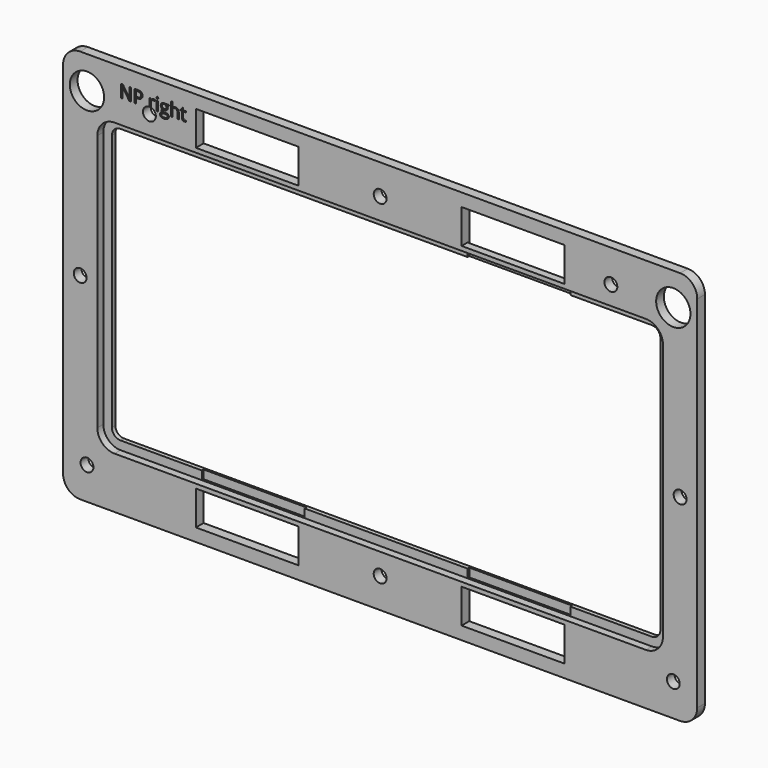
from build123d import *

# Parameters (mm, degrees)
F0_R         = 2.38125
F0_W         = 38.1
F0_H         = 12.7
F0_R_2       = 6.35
F0_R_3       = 2.3876
F1_DEPTH     = 0.79375
F3_DEPTH     = 3.571875
F4_W         = 38.1
F4_H         = 6.4444152495
F4_H_2       = 7.2760339895
F5_DEPTH     = 0.79375
F6_DEPTH     = 0.79375
F7_TEXT_SIZE = 6.5434620612
F8_DEPTH     = 0.396875


# Not quite as in the source:
# - Text() gives the source's letters only with a copy of the font that has no kerning and outlines rounded to 1/6400 em; it was checked with that copy


with BuildPart() as f1:
    # F0 (on Front) → F1 (new body)
    with BuildSketch(Plane.XZ):
        with BuildLine():
            Line((58.8975986641, 62.01647109), (-163.3524013359, 62.01647109))
            ThreePointArc((-163.3524013359, 62.01647109), (-167.8425293965, 60.1565991505), (-169.7024013359, 55.66647109))
            Line((-169.7024013359, 55.66647109), (-169.7024013359, -77.68352891))
            ThreePointArc((-169.7024013359, -77.68352891), (-167.8425293965, -82.1736569705), (-163.3524013359, -84.03352891))
            Line((-163.3524013359, -84.03352891), (58.8975986641, -84.03352891))
            ThreePointArc((58.8975986641, -84.03352891), (63.3877267246, -82.1736569705), (65.2475986641, -77.68352891))
            Line((65.2475986641, -77.68352891), (65.2475986641, 55.66647109))
            ThreePointArc((65.2475986641, 55.66647109), (63.3877267246, 60.1565991505), (58.8975986641, 62.01647109))
        make_face()
        with Locations((-160.8349653662, -71.9910929403)):
            Circle(F0_R, mode=Mode.SUBTRACT)
        with Locations((-101.4399013359, -72.92102891)):
            Rectangle(F0_W, F0_H, mode=Mode.SUBTRACT)
        with Locations((-52.2274013359, -72.92102891)):
            Circle(F0_R, mode=Mode.SUBTRACT)
        with Locations((-3.0149013359, -72.92102891)):
            Rectangle(F0_W, F0_H, mode=Mode.SUBTRACT)
        with Locations((56.3801626943, -71.9910929403)):
            Circle(F0_R, mode=Mode.SUBTRACT)
        with Locations((-163.3524013359, -11.00852891)):
            Circle(F0_R, mode=Mode.SUBTRACT)
        with BuildLine():
            ThreePointArc((-157.0024013359, 36.61647109), (-155.1425293965, 41.1065991505), (-150.6524013359, 42.96647109))
            Line((-150.6524013359, 42.96647109), (46.1975986641, 42.96647109))
            ThreePointArc((46.1975986641, 42.96647109), (50.6877267246, 41.1065991505), (52.5475986641, 36.61647109))
            Line((52.5475986641, 36.61647109), (52.5475986641, -58.63352891))
            ThreePointArc((52.5475986641, -58.63352891), (50.6877267246, -63.1236569705), (46.1975986641, -64.98352891))
            Line((46.1975986641, -64.98352891), (-150.6524013359, -64.98352891))
            ThreePointArc((-150.6524013359, -64.98352891), (-155.1425293965, -63.1236569705), (-157.0024013359, -58.63352891))
            Line((-157.0024013359, -58.63352891), (-157.0024013359, 36.61647109))
        make_face(mode=Mode.SUBTRACT)
        with Locations((-160.8349653662, 49.9740351203)):
            Circle(F0_R_2, mode=Mode.SUBTRACT)
        with Locations((-137.7049037359, 49.9740351203)):
            Circle(F0_R_3, mode=Mode.SUBTRACT)
        with Locations((-101.4399013359, 50.90397109)):
            Rectangle(F0_W, F0_H, mode=Mode.SUBTRACT)
        with Locations((-52.2274013359, 50.90397109)):
            Circle(F0_R, mode=Mode.SUBTRACT)
        with Locations((58.8975986641, -11.00852891)):
            Circle(F0_R, mode=Mode.SUBTRACT)
        with Locations((-3.0149013359, 50.90397109)):
            Rectangle(F0_W, F0_H, mode=Mode.SUBTRACT)
        with Locations((33.2501010641, 49.9740351203)):
            Circle(F0_R_3, mode=Mode.SUBTRACT)
        with Locations((56.3801626943, 49.9740351203)):
            Circle(F0_R_2, mode=Mode.SUBTRACT)
        with BuildLine():
            Line((46.1975986641, 42.96647109), (-150.6524013359, 42.96647109))
            ThreePointArc((-150.6524013359, 42.96647109), (-155.1425293965, 41.1065991505), (-157.0024013359, 36.61647109))
            Line((-157.0024013359, 36.61647109), (-157.0024013359, -58.63352891))
            ThreePointArc((-157.0024013359, -58.63352891), (-155.1425293965, -63.1236569705), (-150.6524013359, -64.98352891))
            Line((-150.6524013359, -64.98352891), (46.1975986641, -64.98352891))
            ThreePointArc((46.1975986641, -64.98352891), (50.6877267246, -63.1236569705), (52.5475986641, -58.63352891))
            Line((52.5475986641, -58.63352891), (52.5475986641, 36.61647109))
            ThreePointArc((52.5475986641, 36.61647109), (50.6877267246, 41.1065991505), (46.1975986641, 42.96647109))
        make_face()
        with BuildLine():
            ThreePointArc((-153.8274013359, 36.61647109), (-152.8974653662, 38.8615351203), (-150.6524013359, 39.79147109))
            Line((-150.6524013359, 39.79147109), (46.1975986641, 39.79147109))
            ThreePointArc((46.1975986641, 39.79147109), (48.4426626943, 38.8615351203), (49.3725986641, 36.61647109))
            Line((49.3725986641, 36.61647109), (49.3725986641, -58.63352891))
            ThreePointArc((49.3725986641, -58.63352891), (48.4426626943, -60.8785929403), (46.1975986641, -61.80852891))
            Line((46.1975986641, -61.80852891), (-150.6524013359, -61.80852891))
            ThreePointArc((-150.6524013359, -61.80852891), (-152.8974653662, -60.8785929403), (-153.8274013359, -58.63352891))
            Line((-153.8274013359, -58.63352891), (-153.8274013359, 36.61647109))
        make_face(mode=Mode.SUBTRACT)
    extrude(amount=F1_DEPTH)

    # F0 (on Front) → F3 (join)
    with BuildSketch(Plane.XZ):
        with BuildLine():
            Line((58.8975986641, 62.01647109), (-163.3524013359, 62.01647109))
            ThreePointArc((-163.3524013359, 62.01647109), (-167.8425293965, 60.1565991505), (-169.7024013359, 55.66647109))
            Line((-169.7024013359, 55.66647109), (-169.7024013359, -77.68352891))
            ThreePointArc((-169.7024013359, -77.68352891), (-167.8425293965, -82.1736569705), (-163.3524013359, -84.03352891))
            Line((-163.3524013359, -84.03352891), (58.8975986641, -84.03352891))
            ThreePointArc((58.8975986641, -84.03352891), (63.3877267246, -82.1736569705), (65.2475986641, -77.68352891))
            Line((65.2475986641, -77.68352891), (65.2475986641, 55.66647109))
            ThreePointArc((65.2475986641, 55.66647109), (63.3877267246, 60.1565991505), (58.8975986641, 62.01647109))
        make_face()
        with Locations((-160.8349653662, -71.9910929403)):
            Circle(F0_R, mode=Mode.SUBTRACT)
        with Locations((-101.4399013359, -72.92102891)):
            Rectangle(F0_W, F0_H, mode=Mode.SUBTRACT)
        with Locations((-52.2274013359, -72.92102891)):
            Circle(F0_R, mode=Mode.SUBTRACT)
        with Locations((-3.0149013359, -72.92102891)):
            Rectangle(F0_W, F0_H, mode=Mode.SUBTRACT)
        with Locations((56.3801626943, -71.9910929403)):
            Circle(F0_R, mode=Mode.SUBTRACT)
        with Locations((-163.3524013359, -11.00852891)):
            Circle(F0_R, mode=Mode.SUBTRACT)
        with BuildLine():
            ThreePointArc((-157.0024013359, 36.61647109), (-155.1425293965, 41.1065991505), (-150.6524013359, 42.96647109))
            Line((-150.6524013359, 42.96647109), (46.1975986641, 42.96647109))
            ThreePointArc((46.1975986641, 42.96647109), (50.6877267246, 41.1065991505), (52.5475986641, 36.61647109))
            Line((52.5475986641, 36.61647109), (52.5475986641, -58.63352891))
            ThreePointArc((52.5475986641, -58.63352891), (50.6877267246, -63.1236569705), (46.1975986641, -64.98352891))
            Line((46.1975986641, -64.98352891), (-150.6524013359, -64.98352891))
            ThreePointArc((-150.6524013359, -64.98352891), (-155.1425293965, -63.1236569705), (-157.0024013359, -58.63352891))
            Line((-157.0024013359, -58.63352891), (-157.0024013359, 36.61647109))
        make_face(mode=Mode.SUBTRACT)
        with Locations((-160.8349653662, 49.9740351203)):
            Circle(F0_R_2, mode=Mode.SUBTRACT)
        with Locations((-137.7049037359, 49.9740351203)):
            Circle(F0_R_3, mode=Mode.SUBTRACT)
        with Locations((-101.4399013359, 50.90397109)):
            Rectangle(F0_W, F0_H, mode=Mode.SUBTRACT)
        with Locations((-52.2274013359, 50.90397109)):
            Circle(F0_R, mode=Mode.SUBTRACT)
        with Locations((58.8975986641, -11.00852891)):
            Circle(F0_R, mode=Mode.SUBTRACT)
        with Locations((-3.0149013359, 50.90397109)):
            Rectangle(F0_W, F0_H, mode=Mode.SUBTRACT)
        with Locations((33.2501010641, 49.9740351203)):
            Circle(F0_R_3, mode=Mode.SUBTRACT)
        with Locations((56.3801626943, 49.9740351203)):
            Circle(F0_R_2, mode=Mode.SUBTRACT)
    extrude(amount=F3_DEPTH)

    # F4 (on face) → F5 (cut)
    with BuildSketch(Plane(origin=(0, 0, 0), x_dir=(-1, 0, 0), z_dir=(0, 1, 0))):
        with Locations((3.0149013359, 41.3317634652)):
            Rectangle(F4_W, F4_H)
        with Locations((3.0149013359, -62.9330119152)):
            Rectangle(F4_W, F4_H_2)
        with Locations((101.4399013359, -62.9330119152)):
            Rectangle(F4_W, F4_H_2)
    extrude(amount=-F5_DEPTH, mode=Mode.SUBTRACT)

    # F2 (on face) → F6 (join)
    with BuildSketch(Plane.XZ):
        with BuildLine():
            Line((46.1975986641, 42.96647109), (-150.6524013359, 42.96647109))
            ThreePointArc((-150.6524013359, 42.96647109), (-155.1425293965, 41.1065991505), (-157.0024013359, 36.61647109))
            Line((-157.0024013359, 36.61647109), (-157.0024013359, -58.63352891))
            ThreePointArc((-157.0024013359, -58.63352891), (-155.1425293965, -63.1236569705), (-150.6524013359, -64.98352891))
            Line((-150.6524013359, -64.98352891), (46.1975986641, -64.98352891))
            ThreePointArc((46.1975986641, -64.98352891), (50.6877267246, -63.1236569705), (52.5475986641, -58.63352891))
            Line((52.5475986641, -58.63352891), (52.5475986641, 36.61647109))
            ThreePointArc((52.5475986641, 36.61647109), (50.6877267246, 41.1065991505), (46.1975986641, 42.96647109))
        make_face()
        with BuildLine():
            ThreePointArc((46.1975986641, 39.79147109), (48.4426626943, 38.8615351203), (49.3725986641, 36.61647109))
            Line((49.3725986641, 36.61647109), (49.3725986641, -58.63352891))
            ThreePointArc((49.3725986641, -58.63352891), (48.4426626943, -60.8785929403), (46.1975986641, -61.80852891))
            Line((46.1975986641, -61.80852891), (-150.6524013359, -61.80852891))
            ThreePointArc((-150.6524013359, -61.80852891), (-152.8974653662, -60.8785929403), (-153.8274013359, -58.63352891))
            Line((-153.8274013359, -58.63352891), (-153.8274013359, 36.61647109))
            ThreePointArc((-153.8274013359, 36.61647109), (-152.8974653662, 38.8615351203), (-150.6524013359, 39.79147109))
            Line((-150.6524013359, 39.79147109), (46.1975986641, 39.79147109))
        make_face(mode=Mode.SUBTRACT)
    extrude(amount=-F6_DEPTH)

    # F7 (on face) → F8 (cut)
    with BuildSketch(Plane.XZ.offset(3.571875)):
        with Locations((-148.8088667393, 51.7694167793)):
            Text('NP right', F7_TEXT_SIZE, font='Open Sans', text_align=(TextAlign.LEFT, TextAlign.BOTTOM))
    extrude(amount=-F8_DEPTH, mode=Mode.SUBTRACT)


solid = f1.part
